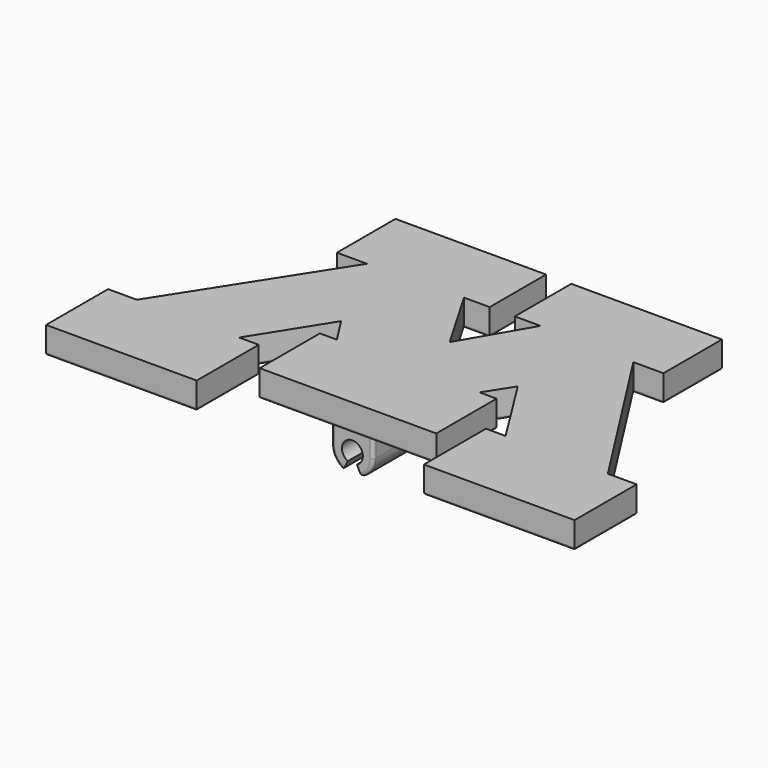
from build123d import *

# Parameters (mm, degrees)
F0_R     = 1
F1_DEPTH = 5
F3_DEPTH = 10.001
F4_R     = 0.3
F6_DEPTH = 2.54
F7_R     = 0.2


with BuildPart() as f1:
    # F0 (on Front) → F1 (new body, symmetric)
    with BuildSketch(Plane.XZ):
        with BuildLine():
            Line((-2, 2), (-2, 0))
            ThreePointArc((-2, 0), (0, -2), (2, 0))
            Line((2, 0), (2, 2))
            Line((2, 2), (0, 2))
            Line((0, 2), (-2, 2))
        make_face()
        Circle(F0_R, mode=Mode.SUBTRACT)
    extrude(amount=F1_DEPTH, both=True)

    # F2 (on face) → F3 (cut, through all)
    with BuildSketch(Plane.XZ.offset(5)):
        with BuildLine():
            Line((0.875, -1.7984368212), (0, 0))
            Line((0, 0), (-0.875, -1.7984368212))
            ThreePointArc((-0.875, -1.7984368212), (0, -2), (0.875, -1.7984368212))
        make_face()
    extrude(amount=-F3_DEPTH, mode=Mode.SUBTRACT)

    # F4
    f4_edges = [f1.edges().sort_by_distance(p)[0] for p in [
        (-0.875, 0, -1.798437),
        (0.875, 0, -1.798437),
        (-1.695582, -5, -1.06066),
        (-2, -5, 1),
        (1.695582, -5, -1.06066),
        (1.695582, 5, -1.06066),
        (2, 5, 1),
        (-1.695582, 5, -1.06066),
        (-2, 5, 1),
        (2, -5, 1),
    ]]
    fillet(f4_edges, radius=F4_R)

    # F5 (on face) → F6 (join)
    with BuildSketch(Plane.XY.offset(2)):
        Polygon((-1.2036230182, 19.6684543043), (-15.6138911843, 19.6684543043), (-15.6138911843, 12.6715609804), (-12.7401659265, 12.6715609804), (-22.5274879485, -2.6133179199), (-25.2762660384, -2.6133179199), (-25.2762660384, -10.0266933441), (-10.8659984544, -10.0266933441), (-10.8659984544, -2.6133179199), (-12.7401659265, -2.6133179199), (-8.4504038095, 4.2169820517), (-6.826125551, 1.676443615), (-8.4504038095, 1.676443615), (-8.4504038095, -5.5286907591), (0, -5.5286907591), (8.4504038095, -5.5286907591), (8.4504038095, 1.676443615), (6.826125551, 1.676443615), (8.4504038095, 4.2169820517), (12.7401659265, -2.6133179199), (10.8659984544, -2.6133179199), (10.8659984544, -10.0266933441), (25.2762660384, -10.0266933441), (25.2762660384, -2.6133179199), (22.5274879485, -2.6133179199), (12.7401659265, 12.6715609804), (15.6138911843, 12.6715609804), (15.6138911843, 19.6684543043), (1.2036230182, 19.6684543043), (1.2036230182, 12.9214497283), (3.6608641967, 12.9214497283), (0, 6.6325762309), (-3.6608641967, 12.9214497283), (-1.2036230182, 12.9214497283), align=None)
        with BuildLine():
            Line((2, 4.7), (2, -4.7))
            ThreePointArc((2, -4.7), (1.9121320344, -4.9121320344), (1.7, -5))
            Line((1.7, -5), (-1.7, -5))
            ThreePointArc((-1.7, -5), (-1.9121320344, -4.9121320344), (-2, -4.7))
            Line((-2, -4.7), (-2, 4.7))
            ThreePointArc((-2, 4.7), (-1.9121320344, 4.9121320344), (-1.7, 5))
            Line((-1.7, 5), (1.7, 5))
            ThreePointArc((1.7, 5), (1.9121320344, 4.9121320344), (2, 4.7))
        make_face(mode=Mode.SUBTRACT)
        with BuildLine():
            ThreePointArc((1.7, -5), (1.9121320344, -4.9121320344), (2, -4.7))
            Line((2, -4.7), (2, 4.7))
            ThreePointArc((2, 4.7), (1.9121320344, 4.9121320344), (1.7, 5))
            Line((1.7, 5), (-1.7, 5))
            ThreePointArc((-1.7, 5), (-1.9121320344, 4.9121320344), (-2, 4.7))
            Line((-2, 4.7), (-2, -4.7))
            ThreePointArc((-2, -4.7), (-1.9121320344, -4.9121320344), (-1.7, -5))
            Line((-1.7, -5), (1.7, -5))
        make_face()
    extrude(amount=F6_DEPTH)

    # F7
    f7_edges = [f1.edges().sort_by_distance(p)[0] for p in [
        (14.177029, 12.671561, 2),
        (17.633827, 5.029122, 2),
        (15.613891, 16.170008, 2),
        (23.901877, -2.613318, 2),
        (8.408757, 19.668454, 2),
        (25.276266, -6.320006, 2),
        (1.203623, 16.294952, 2),
        (18.071132, -10.026693, 2),
        (2.432244, 12.92145, 2),
        (10.865998, -6.320006, 2),
        (1.830432, 9.777013, 2),
        (11.803082, -2.613318, 2),
        (-1.830432, 9.777013, 2),
        (10.595285, 0.801832, 2),
        (-2.432244, 12.92145, 2),
        (7.638265, 2.946713, 2),
        (-1.203623, 16.294952, 2),
        (7.638265, 1.676444, 2),
        (-8.408757, 19.668454, 2),
        (8.450404, -1.926124, 2),
        (-15.613891, 16.170008, 2),
        (0, -5.528691, 2),
        (-14.177029, 12.671561, 2),
        (-8.450404, -1.926124, 2),
        (-17.633827, 5.029122, 2),
        (-7.638265, 1.676444, 2),
        (-23.901877, -2.613318, 2),
        (-7.638265, 2.946713, 2),
        (-25.276266, -6.320006, 2),
        (-10.595285, 0.801832, 2),
        (-18.071132, -10.026693, 2),
        (-11.803082, -2.613318, 2),
        (-10.865998, -6.320006, 2),
        (1.912132, 4.912132, 2),
        (0, 5, 2),
        (-1.912132, 4.912132, 2),
        (-2, 0, 2),
        (-1.912132, -4.912132, 2),
        (0, -5, 2),
        (1.912132, -4.912132, 2),
        (2, 0, 2),
    ]]
    fillet(f7_edges, radius=F7_R)


solid = f1.part
